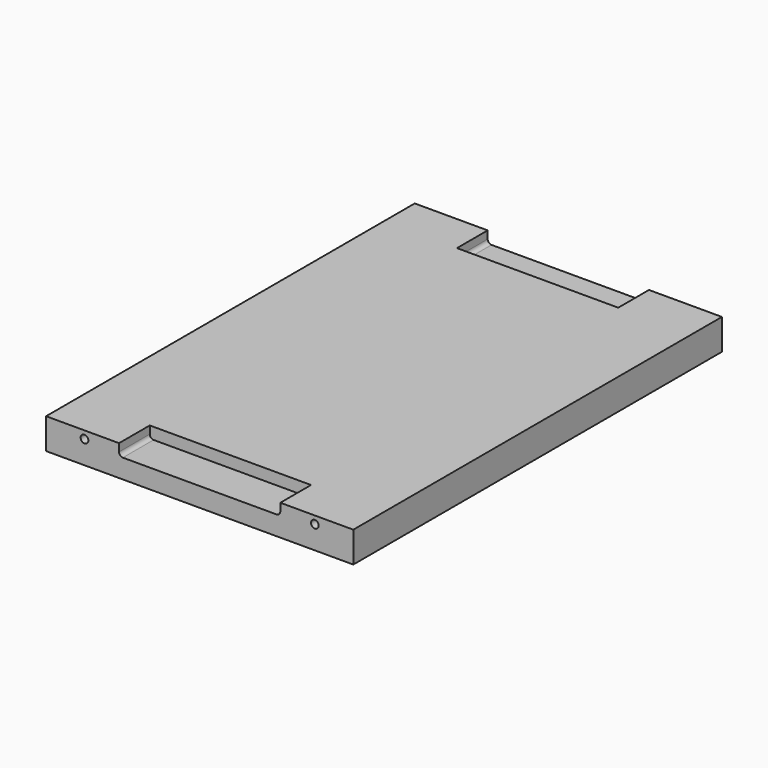
from build123d import *

# Parameters (mm, degrees)
F0_W     = 50.8
F0_H     = 5.08
F1_DEPTH = 38.1
F2_R     = 0.635
F3_DEPTH = 6.35


# Not quite as in the source:
# - a pattern or mirror of a feature is missing from the dataset's text; its kind, count and spacing are read off the source's solid


with BuildPart() as f1:
    # F0 (on Front) → F1 (new body, symmetric)
    with BuildSketch(Plane.XZ):
        Rectangle(F0_W, F0_H)
    extrude(amount=F1_DEPTH, both=True)

    # F2 (on face) → F3 (cut)
    with BuildSketch(Plane.XZ.offset(38.1)):
        with Locations((-19.05, 1.27)):
            Circle(F2_R)
        with BuildLine():
            ThreePointArc((-13.335, 1.27), (-13.1490128061, 0.8209871939), (-12.7, 0.635))
            Line((-12.7, 0.635), (0, 0.635))
            Line((0, 0.635), (12.7, 0.635))
            ThreePointArc((12.7, 0.635), (13.1490128061, 0.8209871939), (13.335, 1.27))
            Line((13.335, 1.27), (13.335, 2.54))
            Line((13.335, 2.54), (-13.335, 2.54))
            Line((-13.335, 2.54), (-13.335, 1.27))
        make_face()
        with Locations((19.05, 1.27)):
            Circle(F2_R)
    f3 = extrude(amount=-F3_DEPTH, mode=Mode.SUBTRACT)

    # F3_copies: F3 across plane
    add(f3.mirror(Plane.ZX), mode=Mode.SUBTRACT)


solid = f1.part
